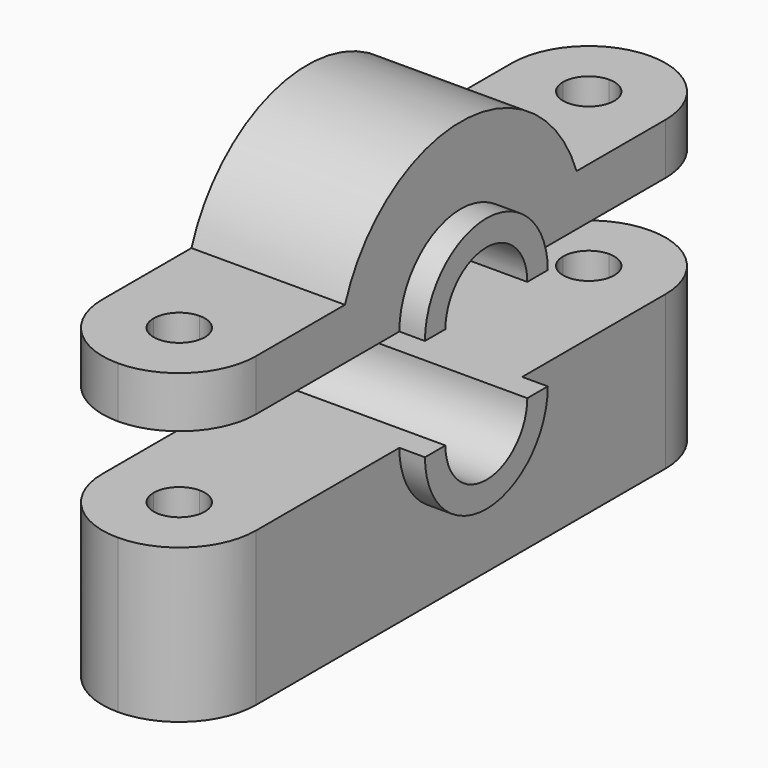
from build123d import *

# Parameters (mm, degrees)
F1_DEPTH = 20
F0_W     = 10
F0_H     = 10
F2_DEPTH = 15
F0_H_2   = 30
F3_DEPTH = 5
F4_R     = 4.99999
F4_2_R   = 4.99999
F5_R     = 14.99999
F5_2_R   = 14.99999


# Not quite as in the source:
# - a fillet or chamfer is up to 0.001 mm smaller than in the source, because OpenCascade refuses the exact size


with BuildPart() as f1:
    # F0 (on Right) → F1 (new body, symmetric)
    with BuildSketch(Plane.YZ):
        with BuildLine():
            Line((-15, 50), (-10, 50))
            ThreePointArc((-10, 50), (0, 60), (10, 50))
            Line((10, 50), (15, 50))
            ThreePointArc((15, 50), (0, 65), (-15, 50))
        make_face()
    extrude(amount=F1_DEPTH, both=True)

    # F0 (on Right) → F2 (join, symmetric)
    with BuildSketch(Plane.YZ):
        with Locations((-60, 55)):
            Rectangle(F0_W, F0_H)
        with BuildLine():
            Line((-45, 50), (-15, 50))
            ThreePointArc((-15, 50), (0, 65), (15, 50))
            Line((15, 50), (45, 50))
            Line((45, 50), (45, 60))
            Line((45, 60), (28.2842712475, 60))
            ThreePointArc((28.2842712475, 60), (0, 80), (-28.2842712475, 60))
            Line((-28.2842712475, 60), (-45, 60))
            Line((-45, 60), (-45, 50))
        make_face()
        with Locations((-50, 55)):
            Rectangle(F0_W, F0_H)
        with Locations((50, 55)):
            Rectangle(F0_W, F0_H)
        with Locations((60, 55)):
            Rectangle(F0_W, F0_H)
    extrude(amount=F2_DEPTH, both=True)


with BuildPart() as f1b:
    # F0 (on Right) → F1, piece 2 (new body, symmetric)
    with BuildSketch(Plane.YZ):
        with BuildLine():
            Line((-10, 30), (-15, 30))
            ThreePointArc((-15, 30), (0, 15), (15, 30))
            Line((15, 30), (10, 30))
            ThreePointArc((10, 30), (0, 20), (-10, 30))
        make_face()
    extrude(amount=F1_DEPTH, both=True)

    # F0 (on Right) → F2, piece 2 (join, symmetric)
    with BuildSketch(Plane.YZ):
        with BuildLine():
            Line((-45, 30), (-45, 0))
            Line((-45, 0), (0, 0))
            Line((0, 0), (45, 0))
            Line((45, 0), (45, 30))
            Line((45, 30), (15, 30))
            ThreePointArc((15, 30), (0, 15), (-15, 30))
            Line((-15, 30), (-45, 30))
        make_face()
        Polygon((45, 30), (45, 0), (50, 0), (55, 0), (55, 30), (50, 30), align=None)
        with Locations((60, 15)):
            Rectangle(F0_W, F0_H_2)
        Polygon((-55, 30), (-55, 0), (-50, 0), (-45, 0), (-45, 30), (-50, 30), align=None)
        with Locations((-60, 15)):
            Rectangle(F0_W, F0_H_2)
    extrude(amount=F2_DEPTH, both=True)


with BuildPart() as f3_tool:
    # F0 (on Right) → F3 (new body, symmetric)
    with BuildSketch(Plane.YZ):
        with Locations((-50, 55)):
            Rectangle(F0_W, F0_H)
        Polygon((-55, 30), (-55, 0), (-50, 0), (-45, 0), (-45, 30), (-50, 30), align=None)
        with Locations((50, 55)):
            Rectangle(F0_W, F0_H)
        Polygon((45, 30), (45, 0), (50, 0), (55, 0), (55, 30), (50, 30), align=None)
    extrude(amount=F3_DEPTH, both=True)


with BuildPart() as f1_1:
    add(f1.part)

    # F3: cut by f3_tool
    add(f3_tool.part, mode=Mode.SUBTRACT)

    # F4 (radius 5 in the source; OpenCascade refuses exactly that, so slightly less here)
    f4_edges = [f1_1.edges().sort_by_distance(p)[0] for p in [
        (-5, -45, 55),
        (-5, 55, 55),
        (-5, -55, 55),
        (-5, 45, 55),
        (5, -55, 55),
        (5, 45, 55),
        (5, 55, 55),
        (5, -45, 55),
    ]]
    fillet(f4_edges, radius=F4_R)

    # F5#2 (radius 15 in the source; OpenCascade refuses exactly that, so slightly less here)
    f5_2_edges = [f1_1.edges().sort_by_distance(p)[0] for p in [
        (-15, -65, 55),
        (15, -65, 55),
        (15, 65, 55),
        (-15, 65, 55),
    ]]
    fillet(f5_2_edges, radius=F5_2_R)


with BuildPart() as f1b_1:
    add(f1b.part)

    # F3: cut by f3_tool
    add(f3_tool.part, mode=Mode.SUBTRACT)

    # F4#2 (radius 5 in the source; OpenCascade refuses exactly that, so slightly less here)
    f4_2_edges = [f1b_1.edges().sort_by_distance(p)[0] for p in [
        (-5, 55, 15),
        (-5, -45, 15),
        (-5, -55, 15),
        (-5, 45, 15),
        (5, -55, 15),
        (5, -45, 15),
        (5, 55, 15),
        (5, 45, 15),
    ]]
    fillet(f4_2_edges, radius=F4_2_R)

    # F5 (radius 15 in the source; OpenCascade refuses exactly that, so slightly less here)
    f5_edges = [f1b_1.edges().sort_by_distance(p)[0] for p in [
        (15, -65, 15),
        (-15, -65, 15),
        (15, 65, 15),
        (-15, 65, 15),
    ]]
    fillet(f5_edges, radius=F5_R)


solid = Compound([f1_1.part, f1b_1.part])
